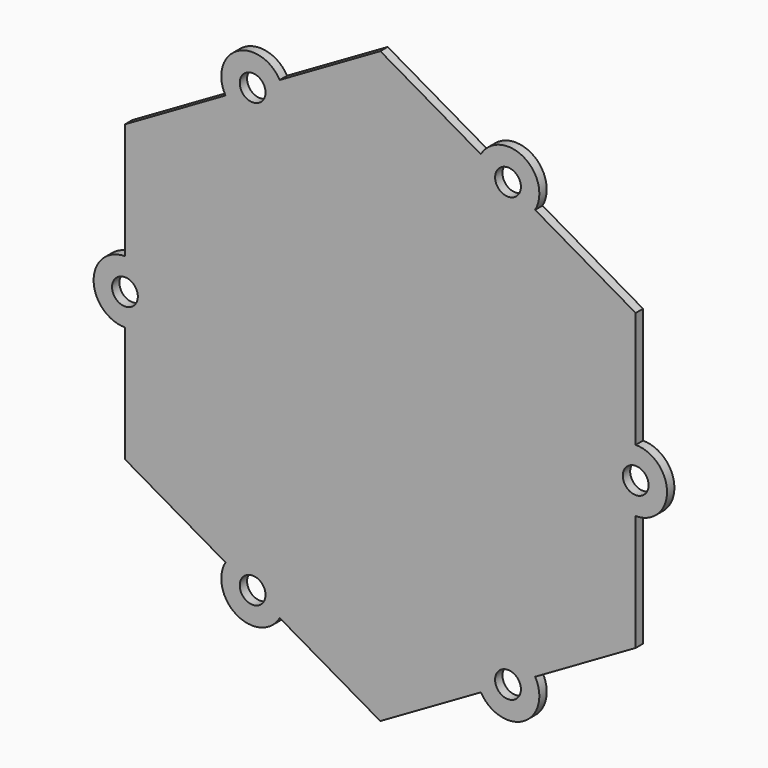
from build123d import *

# Parameters (mm, degrees)
F1_DEPTH = 3.175
F4_DEPTH = 3.175
F5_R     = 4.445
F6_DEPTH = 3.176


# Not quite as in the source:
# - a length typed as a fraction of an inch, garbled in the dataset ("3 / 203.2 mm" for 3/8 in), is restored


with BuildPart() as f1:
    # F0 (on Front) → F1 (new body)
    with BuildSketch(Plane.XZ):
        Polygon((87.9881810245, 50.8), (0, 101.6), (-87.9881810245, 50.8), (-87.9881810245, -50.8), (0, -101.6), (87.9881810245, -50.8), align=None)
    extrude(amount=F1_DEPTH)

    # F3 (on Front) → F4 (join)
    with BuildSketch(Plane.XZ):
        with BuildLine():
            ThreePointArc((87.9881810245, -10.795), (98.7831810245, 0), (87.9881810245, 10.795))
            Line((87.9881810245, 10.795), (87.9881810245, -10.795))
        make_face()
        with BuildLine():
            Line((34.6453462784, 81.5975), (53.3428347461, 70.8025))
            ThreePointArc((53.3428347461, 70.8025), (49.3915905122, 85.5487442339), (34.6453462784, 81.5975))
        make_face()
        with BuildLine():
            Line((-53.3428347461, 70.8025), (-34.6453462784, 81.5975))
            ThreePointArc((-34.6453462784, 81.5975), (-49.3915905122, 85.5487442339), (-53.3428347461, 70.8025))
        make_face()
        with BuildLine():
            Line((-87.9881810245, -10.795), (-87.9881810245, 10.795))
            ThreePointArc((-87.9881810245, 10.795), (-98.7831810245, 0), (-87.9881810245, -10.795))
        make_face()
        with BuildLine():
            Line((-34.6453462784, -81.5975), (-53.3428347461, -70.8025))
            ThreePointArc((-53.3428347461, -70.8025), (-49.3915905122, -85.5487442339), (-34.6453462784, -81.5975))
        make_face()
        with BuildLine():
            Line((53.3428347461, -70.8025), (34.6453462784, -81.5975))
            ThreePointArc((34.6453462784, -81.5975), (49.3915905122, -85.5487442339), (53.3428347461, -70.8025))
        make_face()
    extrude(amount=F4_DEPTH)

    # F5 (on face) → F6 (cut, through all)
    with BuildSketch(Plane.XZ.offset(3.175)):
        with Locations((43.9940905122, 76.2)):
            Circle(F5_R)
        with Locations((-43.9940905122, 76.2)):
            Circle(F5_R)
        with Locations((-87.9881810245, 0)):
            Circle(F5_R)
        with Locations((-43.9940905122, -76.2)):
            Circle(F5_R)
        with Locations((43.9940905122, -76.2)):
            Circle(F5_R)
        with Locations((87.9881810245, 0)):
            Circle(F5_R)
    extrude(amount=-F6_DEPTH, mode=Mode.SUBTRACT)


solid = f1.part
